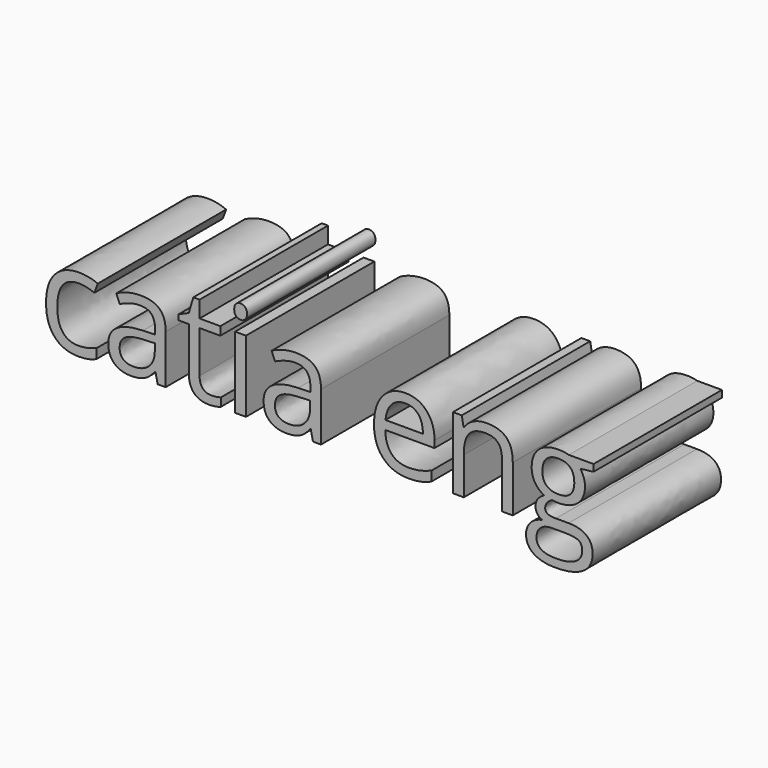
from build123d import *

# Parameters (mm, degrees)
F2_TEXT_SIZE = 85.965424983
F0_DEPTH     = 103.2278109342


# Not quite as in the source:
# - the program builds the solid bodies; features that only make, move or delete a surface that nothing else refers to are left out
# - Text() gives the source's letters only with a copy of the font that has no kerning and outlines rounded to 1/6400 em; it was checked with that copy


with BuildPart() as f0:
    # F2 (on Front) → F0 (new body)
    with BuildSketch(Plane.XZ):
        with Locations((66.8866708875, 26.5051759779)):
            Text('catia eng', F2_TEXT_SIZE, font='Open Sans', text_align=(TextAlign.LEFT, TextAlign.BOTTOM))
    extrude(amount=F0_DEPTH)


solid = f0.part
